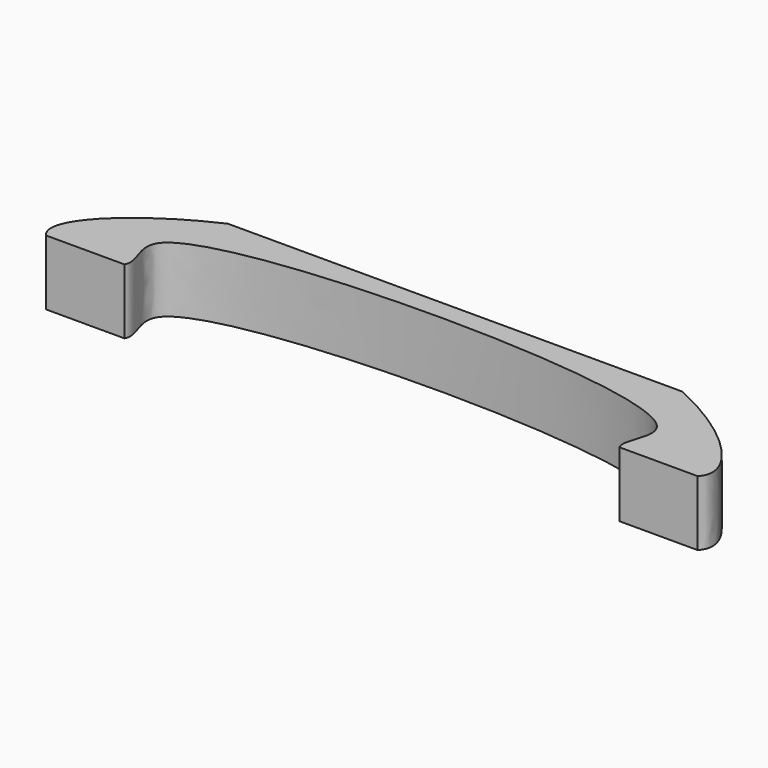
from build123d import *

# Parameters (mm, degrees)
F1_DEPTH = 25


with BuildPart() as f1:
    # F0 (on Top) → F1 (new body)
    with BuildSketch(Plane.XY):
        with BuildLine():
            add(Edge.make_bspline(
                [(-116.2008633957, 0), (-124.3957559353, 8.071296767), (-105.8506085877, 27.534724907), (-78.4516912193, 40)],
                knots=[0, 0, 0, 0, 0.1210513861, 0.1210513861, 0.1210513861, 0.1210513861], degree=3))
            Line((-116.2008633957, 0), (-86.2008633957, 0))
            add(Edge.make_bspline(
                [(103.7991366043, 0), (101.235325492, 4.4215579911), (134.5147878784, 37.1139422067), (-116.9165146698, 37.1139422067), (-83.6370522834, 4.4215579911), (-86.2008633957, 0)],
                knots=[0.5471247269, 0.5471247269, 0.5471247269, 0.5471247269, 0.6163755226, 0.8413468307, 0.9105976264, 0.9105976264, 0.9105976264, 0.9105976264], degree=3))
            Line((103.7991366043, 0), (133.7991366043, 0))
            add(Edge.make_bspline(
                [(96.0499644279, 40), (123.4488817963, 27.534724907), (141.9940291439, 8.071296767), (133.7991366043, 0)],
                knots=[0.3366709672, 0.3366709672, 0.3366709672, 0.3366709672, 0.4577223533, 0.4577223533, 0.4577223533, 0.4577223533], degree=3))
            Line((96.0499644279, 40), (-78.4516912193, 40))
        make_face()
    extrude(amount=F1_DEPTH)


solid = f1.part
